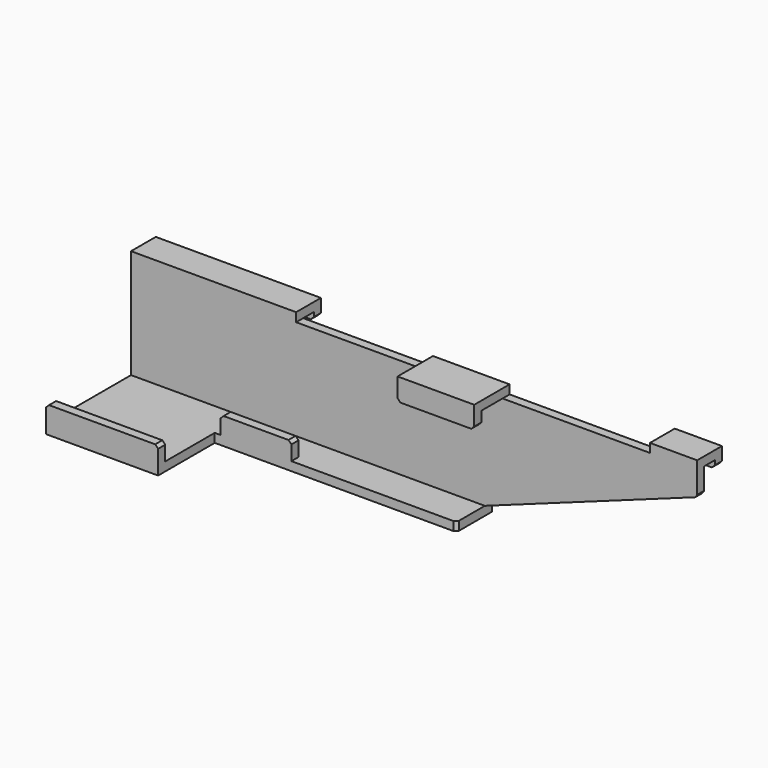
from build123d import *

# Parameters (mm, degrees)
F1_DEPTH      = 19.05
F2_W          = 355.6
F2_H          = 66.675
F2_W_2        = 101.6
F2_W_3        = 165.1
F2_H_2        = 76.2000030398
F3_DEPTH      = 19.05
F4_W          = 101.6
F4_H          = 19.05
F4_W_2        = 355.6
F4_W_3        = 165.1
F5_DEPTH      = 15.875
F6_W          = 241.3
F6_H          = 152.4
F7_DEPTH      = 19.05
F8_W          = 241.3
F8_H          = 19.05
F8_W_2        = 152.4
F9_DEPTH      = 38.1
F10_DEPTH     = 12.7
F11_T1_DEPTH  = 51.7103739472
F11_T3_DEPTH  = 51.7103739472
F11_T5_DEPTH  = 51.7103739472
F11_T7_DEPTH  = 51.7103739472
F11_T9_DEPTH  = 51.7103739472
F11_T11_DEPTH = 42.3922386312


# Not quite as in the source:
# - a fillet or chamfer that OpenCascade refuses, or shapes differently, is made with other operations: its cross-section is extruded or revolved along the edge and cut away or added
# - ends of sketch curves that miss each other by under 0.0002 mm in the source are joined


with BuildPart() as f1:
    # F0 (on Front) → F1 (new body)
    with BuildSketch(Plane.XZ):
        Polygon((1219.2, 0), (0, 0), (0, -215.9), (762, -215.9), (1219.2, -50.8), align=None)
    extrude(amount=F1_DEPTH)

    # F2 (on face) → F3 (join)
    with BuildSketch(Plane.XY):
        with Locations((177.8, 14.2875)):
            Rectangle(F2_W, F2_H)
        with Locations((1168.4, 14.2875)):
            Rectangle(F2_W_2, F2_H)
        with Locations((717.55, -57.1500015199)):
            Rectangle(F2_W_3, F2_H_2)
        Polygon((635, 0), (635, -19.05), (800.1, -19.05), (800.1, -3.0398e-06), (647.7, 0), align=None)
    extrude(amount=F3_DEPTH)

    # F4 (on face) → F5 (join)
    with BuildSketch(Plane.XY):
        with Locations((1168.4, 38.1)):
            Rectangle(F4_W, F4_H)
        with Locations((177.8, 38.1)):
            Rectangle(F4_W_2, F4_H)
        with Locations((717.55, -85.7250030398)):
            Rectangle(F4_W_3, F4_H)
    extrude(amount=-F5_DEPTH)

    # F6 (on face) → F7 (join)
    with BuildSketch(Plane(origin=(0, 0, -215.9), x_dir=(1, 0, 0), z_dir=(0, 0, -1))):
        Polygon((0, 95.25), (0, 0), (762, 0), (762, 95.25), (241.3, 95.25), align=None)
        with Locations((120.65, 171.45)):
            Rectangle(F6_W, F6_H)
    extrude(amount=F7_DEPTH)

    # F8 (on face) → F9 (join)
    with BuildSketch(Plane.XY.offset(-215.9)):
        with Locations((120.65, -238.125)):
            Rectangle(F8_W, F8_H)
        with Locations((330.2, -85.725)):
            Rectangle(F8_W_2, F8_H)
    extrude(amount=F9_DEPTH)

    # F10 (add): a face of the model
    f10_faces = [f1.faces().sort_by_distance(p)[0] for p in [
        (717.55, -85.7250030398, -15.875),
    ]]
    extrude(f10_faces, amount=F10_DEPTH)

    # F11: chamfer of 6.35 on 12 edges, made by hand

    # F11_s2 → F11_t1 (cut)
    with BuildSketch(Plane.XZ.offset(212.2698130264)):
        Polygon((6.35, -177.8), (0, -184.15), (0, -177.8), align=None)
        Polygon((241.3, -184.15), (234.95, -177.8), (241.3, -177.8), align=None)
    extrude(amount=F11_T1_DEPTH, mode=Mode.SUBTRACT)

    # F11_s4 → F11_t3 (cut)
    with BuildSketch(Plane.XZ.offset(59.8698130264)):
        Polygon((260.35, -177.8), (254, -184.15), (254, -177.8), align=None)
        Polygon((406.4, -184.15), (400.05, -177.8), (406.4, -177.8), align=None)
    extrude(amount=F11_T3_DEPTH, mode=Mode.SUBTRACT)

    # F11_s6 → F11_t5 (cut)
    with BuildSketch(Plane.XZ.offset(59.8698160663)):
        Polygon((800.1, -22.225), (793.75, -28.575), (800.1, -28.575), align=None)
        Polygon((635, -22.225), (641.35, -28.575), (635, -28.575), align=None)
    extrude(amount=F11_T5_DEPTH, mode=Mode.SUBTRACT)

    # F11_s8 → F11_t7 (cut)
    with BuildSketch(Plane.XY.offset(-251.2801869736)):
        Polygon((762, -88.9), (755.65, -95.25), (762, -95.25), align=None)
    extrude(amount=F11_T7_DEPTH, mode=Mode.SUBTRACT)

    # F11_s10 → F11_t9 (cut)
    with BuildSketch(Plane.XZ.offset(-63.9551869736)):
        Polygon((1219.2, -9.525), (1212.85, -15.875), (1219.2, -15.875), align=None)
        Polygon((355.6, -9.525), (349.25, -15.875), (355.6, -15.875), align=None)
        Polygon((1117.6, -9.525), (1123.95, -15.875), (1117.6, -15.875), align=None)
        Polygon((0, -9.525), (6.35, -15.875), (0, -15.875), align=None)
    extrude(amount=F11_T9_DEPTH, mode=Mode.SUBTRACT)

    # F11_s12 → F11_t11 (cut)
    with BuildSketch(Plane.XZ.offset(-11.6711193156)):
        Polygon((1219.2, -46.3417146679), (1215.006742345, -52.314231931), (1219.2, -50.8), align=None)
    extrude(amount=F11_T11_DEPTH, mode=Mode.SUBTRACT)


solid = f1.part
